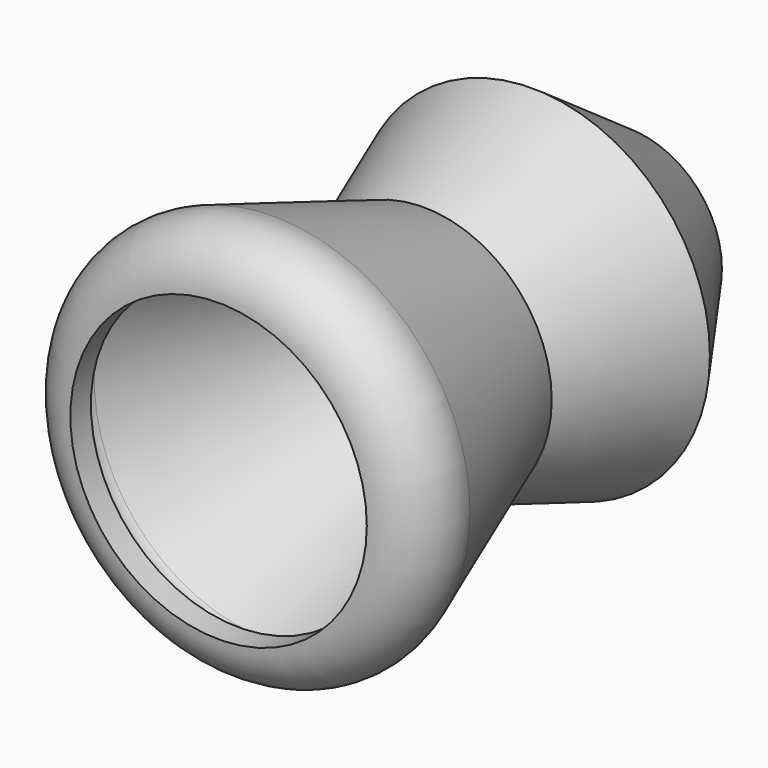
from build123d import *

# Parameters (mm, degrees)
F0_R     = 63.4990492705
F1_DEPTH = 127
F1_TAPER = -20
F2_R     = 25.4
F3_SIZE  = 63.5
F4_T     = -12.7


# Not quite as in the source:
# - a shell that OpenCascade refuses in one call is made with other operations: the cavity is built on its own and cut out


with BuildPart() as f1:
    # F0 (on Front) → F1 (new body, symmetric)
    with BuildSketch(Plane.XZ):
        with Locations((1.6070879065, 0)):
            Circle(F0_R)
    extrude(amount=F1_DEPTH, both=True, taper=F1_TAPER)

    # F2
    f2_edges = [f1.edges().sort_by_distance(p)[0] for p in [
        (-108.116181, -127, 0),
    ]]
    fillet(f2_edges, radius=F2_R)

    # F3
    f3_edges = [f1.edges().sort_by_distance(p)[0] for p in [
        (-108.116181, 127, 0),
    ]]
    chamfer(f3_edges, length=F3_SIZE)

    # F4: a shell. OpenCascade refuses it in one call, so the cavity is built on its own and cut out:
    # the body offset inwards by the wall thickness, plus a prism from it out through each open face.
    f4_core = offset(f1.part, amount=F4_T, kind=Kind.INTERSECTION, mode=Mode.PRIVATE)
    f4_exits = [f4_core.faces().sort_by_distance(p)[0] for p in [
        (1.607088, -114.3, 0),
    ]]
    add(f4_core, mode=Mode.SUBTRACT)
    extrude(f4_exits, amount=-F4_T, mode=Mode.SUBTRACT)


solid = f1.part
